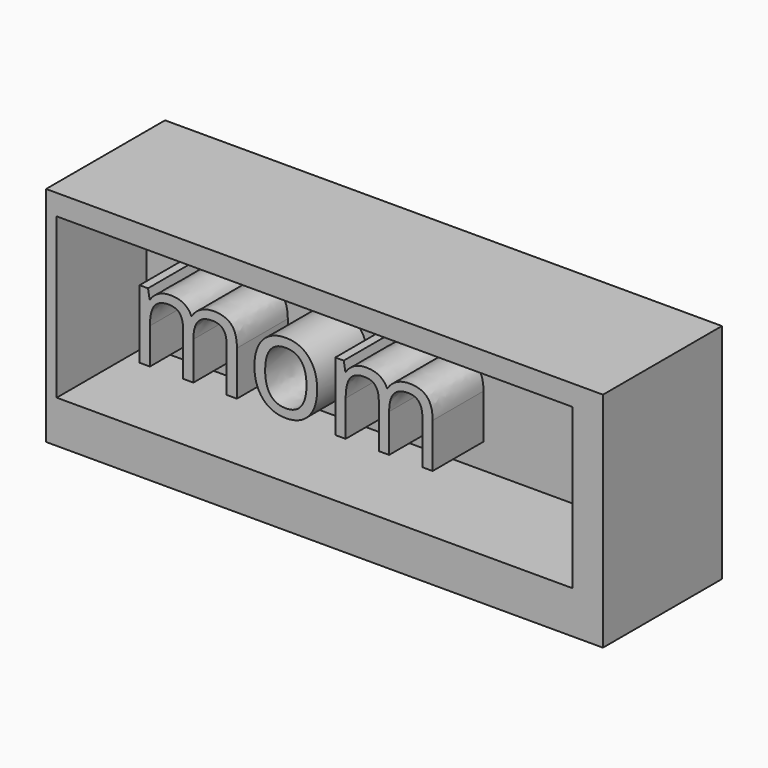
from build123d import *

# Parameters (mm, degrees)
F0_W         = 127
F0_H         = 50.8
F0_W_2       = 117.6311075687
F0_H_2       = 36.4010185003
F1_DEPTH     = 33.9138340205
F2_DEPTH     = 8.3809541538
F3_TEXT_SIZE = 29.0953243772
F4_DEPTH     = 22.8870473802


# Not quite as in the source:
# - Text() gives the source's letters only with a copy of the font that has no kerning and outlines rounded to 1/6400 em; it was checked with that copy


with BuildPart() as f1:
    # F0 (on Front) → F1 (new body)
    with BuildSketch(Plane.XZ):
        with Locations((7.6069384813, -16.3539513917)):
            Rectangle(F0_W, F0_H)
        with Locations((5.3445249796, -13.8675123453)):
            Rectangle(F0_W_2, F0_H_2, mode=Mode.SUBTRACT)
    extrude(amount=F1_DEPTH)

    # F0 (on Front) → F2 (join)
    with BuildSketch(Plane.XZ):
        with Locations((5.3445249796, -13.8675123453)):
            Rectangle(F0_W_2, F0_H_2)
    extrude(amount=F2_DEPTH)


with BuildPart() as f4:
    # F3 (on Front) → F4 (new body)
    with BuildSketch(Plane.XZ):
        with Locations((-45.8941161633, -26.260882616)):
            Text('mom', F3_TEXT_SIZE, font='Open Sans', text_align=(TextAlign.LEFT, TextAlign.BOTTOM))
    extrude(amount=F4_DEPTH)


solid = Compound([f1.part, f4.part])
